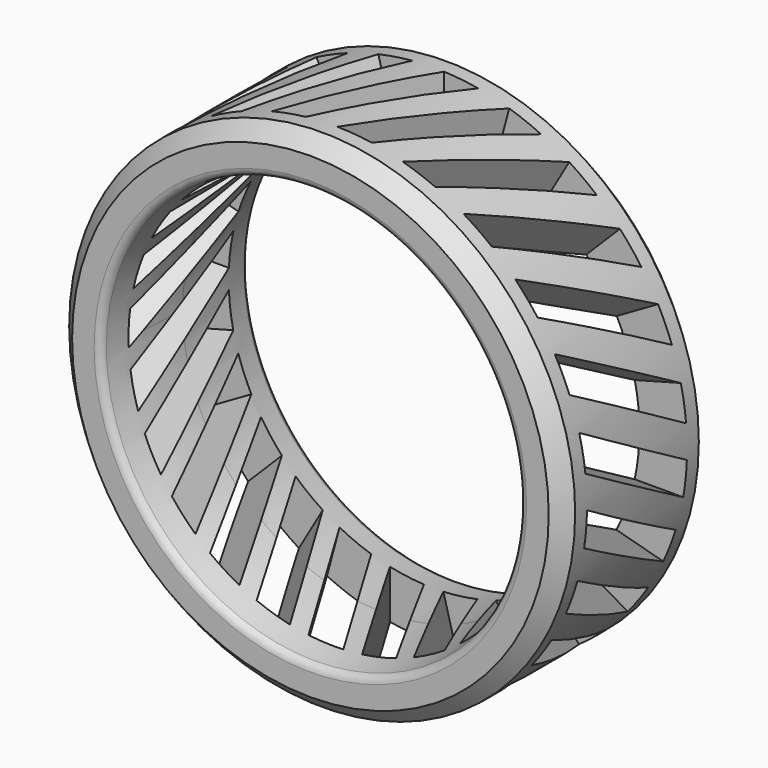
from build123d import *

# Parameters (mm, degrees)
F2_SIZE         = 0.762
F3_R            = 0.381
F6_DEPTH        = 6.35
F6_COPIES_COUNT = 24


# Not quite as in the source:
# - a pattern or mirror of a feature is missing from the dataset's text; its kind, count and spacing are read off the source's solid


with BuildPart() as f1:
    # F0 (on Top) → F1 (revolve)
    with BuildSketch(Plane.XY):
        with BuildLine():
            Line((-13.0996790878, 0), (-10.4267, 0))
            ThreePointArc((-10.4267, 0), (-10.5395705547, 2.3918788461), (-10.8771790878, 4.7625))
            Line((-10.8771790878, 4.7625), (-13.0996790878, 4.7625))
            Line((-13.0996790878, 4.7625), (-13.0996790878, 0))
        make_face()
        with BuildLine():
            ThreePointArc((-10.8771790878, -4.7625), (-10.5395705547, -2.3918788461), (-10.4267, 0))
            Line((-10.4267, 0), (-13.0996790878, 0))
            Line((-13.0996790878, 0), (-13.0996790878, -4.7625))
            Line((-13.0996790878, -4.7625), (-10.8771790878, -4.7625))
        make_face()
    revolve(axis=Axis((0, 6.0321819037, 0), (0, 1, 0)))

    # F2
    f2_edges = [f1.edges().sort_by_distance(p)[0] for p in [
        (13.099679, 4.7625, 0),
        (13.099679, -4.7625, 0),
    ]]
    chamfer(f2_edges, length=F2_SIZE)

    # F3
    f3_edges = [f1.edges().sort_by_distance(p)[0] for p in [
        (10.877179, -4.7625, 0),
        (10.877179, 4.7625, 0),
    ]]
    fillet(f3_edges, radius=F3_R)

    # F5 (on offset) → F6 (cut)
    with BuildSketch(Plane.YZ.offset(15.494)):
        Polygon((3.2385, -2.2815297156), (3.2385, -0.5217660951), (-3.2385, 3.2177315984), (-3.2385, 1.4579679779), align=None)
    f6 = extrude(amount=-F6_DEPTH, mode=Mode.SUBTRACT)

    # F6_copies: F6 ×24 about axis
    f6_copies_axis = Axis((0, 0, 0), (0, 1, 0))
    for i in range(1, F6_COPIES_COUNT):
        add(f6.rotate(f6_copies_axis, i * 360 / F6_COPIES_COUNT), mode=Mode.SUBTRACT)


solid = f1.part
